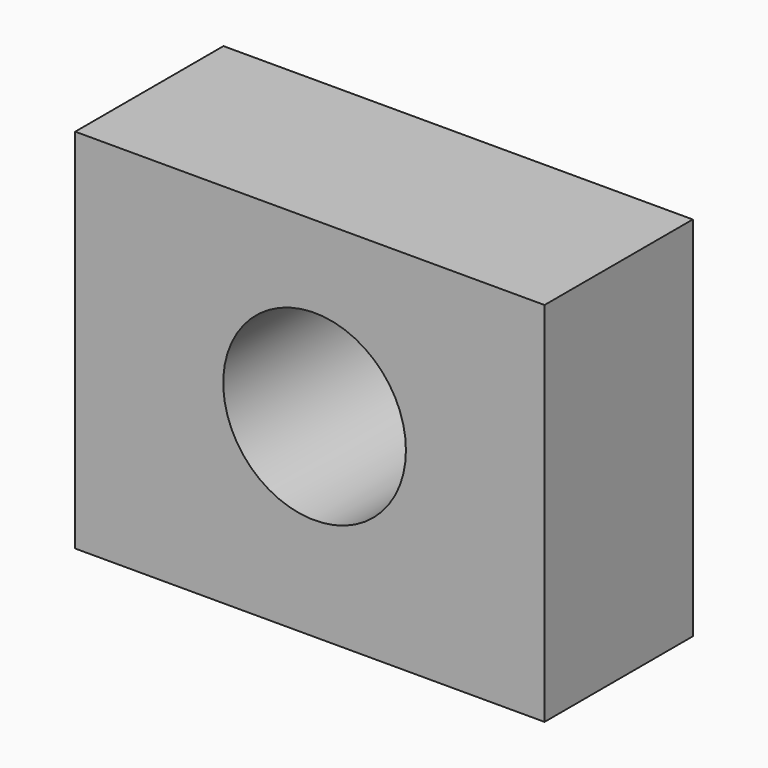
from build123d import *

# Parameters (mm, degrees)
F0_W     = 128.6668404937
F0_H     = 100.6218641996
F0_R     = 25.0442711875
F1_DEPTH = 50.8


# Not quite as in the source:
# - the program builds the solid bodies; features that only make, move or delete a surface that nothing else refers to are left out


with BuildPart() as f1:
    # F0 (on Front) → F1 (new body)
    with BuildSketch(Plane.XZ):
        with Locations((-1.2895353138, -2.8847418725)):
            Rectangle(F0_W, F0_H)
        Circle(F0_R, mode=Mode.SUBTRACT)
    extrude(amount=F1_DEPTH)


solid = f1.part
